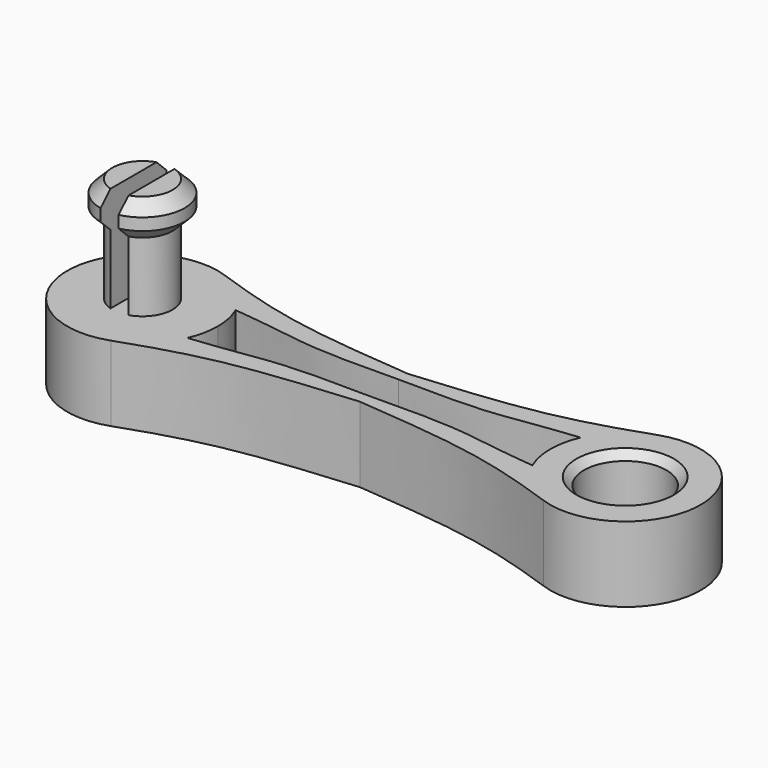
from build123d import *

# Parameters (mm, degrees)
F2_DEPTH = 6.35
F1_W     = 1.778
F1_H     = 3.048
F1_H_2   = 5.842
F1_W_2   = 0.762
F5_DEPTH = 12.7
F6_DEPTH = 2.54


# Not quite as in the source:
# - a pattern or mirror of a feature is missing from the dataset's text; its kind, count and spacing are read off the source's solid
# - a feature names something its author has since deleted; it is built from what else it names


with BuildPart() as f2:
    # F0 (on Top) → F2 (new body)
    with BuildSketch(Plane.XY):
        with BuildLine():
            ThreePointArc((-14.5509208863, -2.5399817128), (-14.1547428746, -1.2973564714), (-14.0208, 0))
            ThreePointArc((-14.0208, 0), (-14.1547428746, 1.2973564714), (-14.5509208863, 2.5399817128))
            ThreePointArc((-14.5509208863, 2.5399817128), (-16.0448887373, 4.6485472727), (-18.2552900028, 5.9872462328))
            ThreePointArc((-18.2552900028, 5.9872462328), (-26.7208, 0), (-18.2552900028, -5.9872462328))
            ThreePointArc((-18.2552900028, -5.9872462328), (-16.0448887373, -4.6485472727), (-14.5509208863, -2.5399817128))
        make_face()
        with BuildLine():
            ThreePointArc((-18.2552900028, 5.9872462328), (-16.0448887373, 4.6485472727), (-14.5509208863, 2.5399817128))
            add(Edge.make_bspline(
                [(0, 1.524), (-9.0764431036, 1.3546369813), (-7.8380626316, 1.8652065321), (-14.5509208863, 2.5399817128)],
                knots=[0, 0, 0, 0, 14.5863469546, 14.5863469546, 14.5863469546, 14.5863469546], degree=3))
            add(Edge.make_bspline(
                [(0, 1.524), (9.0764431036, 1.3546369813), (7.8380626316, 1.8652065321), (14.5509208863, 2.5399817128)],
                knots=[0, 0, 0, 0, 14.5863469546, 14.5863469546, 14.5863469546, 14.5863469546], degree=3))
            ThreePointArc((14.5509208863, 2.5399817128), (16.0448887373, 4.6485472727), (18.2552900028, 5.9872462328))
            add(Edge.make_bspline(
                [(0, 2.54), (8.1250406802, 3.246476237), (11.4529688686, 3.5837408809), (18.2552900028, 5.9872462328)],
                knots=[0, 0, 0, 0, 18.5779202193, 18.5779202193, 18.5779202193, 18.5779202193], degree=3))
            add(Edge.make_bspline(
                [(0, 2.54), (-8.1250406802, 3.246476237), (-11.4529688686, 3.5837408809), (-18.2552900028, 5.9872462328)],
                knots=[0, 0, 0, 0, 18.5779202193, 18.5779202193, 18.5779202193, 18.5779202193], degree=3))
        make_face()
        with BuildLine():
            add(Edge.make_bspline(
                [(0, -1.524), (-9.0764431036, -1.3546369813), (-7.8380626316, -1.8652065321), (-14.5509208863, -2.5399817128)],
                knots=[0, 0, 0, 0, 14.5863469546, 14.5863469546, 14.5863469546, 14.5863469546], degree=3))
            ThreePointArc((-14.5509208863, -2.5399817128), (-16.0448887373, -4.6485472727), (-18.2552900028, -5.9872462328))
            add(Edge.make_bspline(
                [(0, -2.54), (-8.1250406802, -3.246476237), (-11.4529688686, -3.5837408809), (-18.2552900028, -5.9872462328)],
                knots=[0, 0, 0, 0, 18.5779202193, 18.5779202193, 18.5779202193, 18.5779202193], degree=3))
            add(Edge.make_bspline(
                [(0, -2.54), (8.1250406802, -3.246476237), (11.4529688686, -3.5837408809), (18.2552900028, -5.9872462328)],
                knots=[0, 0, 0, 0, 18.5779202193, 18.5779202193, 18.5779202193, 18.5779202193], degree=3))
            ThreePointArc((18.2552900028, -5.9872462328), (16.0448887373, -4.6485472727), (14.5509208863, -2.5399817128))
            add(Edge.make_bspline(
                [(0, -1.524), (9.0764431036, -1.3546369813), (7.8380626316, -1.8652065321), (14.5509208863, -2.5399817128)],
                knots=[0, 0, 0, 0, 14.5863469546, 14.5863469546, 14.5863469546, 14.5863469546], degree=3))
        make_face()
    extrude(amount=F2_DEPTH)

    # F2_copies: F2 across plane


with BuildPart() as f2_1:
    add(f2.part)
    add(f2.part.mirror(Plane(origin=(0, 0, 0), x_dir=(0, 0, 1), z_dir=(1, 0, 0))))

    # F1 (on Front) → F3 (revolve, cut)
    with BuildSketch(Plane.XZ):
        Polygon((20.344351037, 6.35), (20.344351037, 0), (24.459151037, 0), (23.824151037, 0.635), (23.824151037, 5.715), (24.459151037, 6.35), align=None)
    revolve(axis=Axis((20.344351037, 0, 3.175), (0, 0, 1)), mode=Mode.SUBTRACT)

    # F1 (on Front) → F4 (revolve)
    with BuildSketch(Plane.XZ):
        Polygon((-17.8308, 15.24), (-17.8308, 12.192), (-16.8148, 13.208), (-16.8148, 14.224), align=None)
        with Locations((-18.7198, 13.716)):
            Rectangle(F1_W, F1_H)
        with Locations((-22.0218, 13.716)):
            Rectangle(F1_W, F1_H)
        Polygon((-23.9268, 13.208), (-22.9108, 12.192), (-22.9108, 15.24), (-23.9268, 14.224), align=None)
        with Locations((-22.0218, 9.271)):
            Rectangle(F1_W, F1_H_2)
        with Locations((-18.7198, 9.271)):
            Rectangle(F1_W, F1_H_2)
    revolve(axis=Axis((-20.3708, 0, 10.795), (0, 0, 1)))

    # F1 (on Front) → F5 (cut, symmetric)
    with BuildSketch(Plane.XZ):
        with Locations((-19.9898, 13.716)):
            Rectangle(F1_W_2, F1_H)
        with Locations((-20.7518, 13.716)):
            Rectangle(F1_W_2, F1_H)
        with Locations((-19.9898, 9.271)):
            Rectangle(F1_W_2, F1_H_2)
        with Locations((-20.7518, 9.271)):
            Rectangle(F1_W_2, F1_H_2)
    extrude(amount=F5_DEPTH, both=True, mode=Mode.SUBTRACT)

    # F0 (on Top) → F6 (join)
    with BuildSketch(Plane.XY):
        with BuildLine():
            ThreePointArc((-14.5509208863, 2.5399817128), (-14.1547428746, 1.2973564714), (-14.0208, 0))
            ThreePointArc((-14.0208, 0), (-14.1547428746, -1.2973564714), (-14.5509208863, -2.5399817128))
            add(Edge.make_bspline(
                [(0, -1.524), (-9.0764431036, -1.3546369813), (-7.8380626316, -1.8652065321), (-14.5509208863, -2.5399817128)],
                knots=[0, 0, 0, 0, 14.5863469546, 14.5863469546, 14.5863469546, 14.5863469546], degree=3))
            add(Edge.make_bspline(
                [(0, -1.524), (9.0764431036, -1.3546369813), (7.8380626316, -1.8652065321), (14.5509208863, -2.5399817128)],
                knots=[0, 0, 0, 0, 14.5863469546, 14.5863469546, 14.5863469546, 14.5863469546], degree=3))
            ThreePointArc((14.5509208863, -2.5399817128), (14.0208, 0), (14.5509208863, 2.5399817128))
            add(Edge.make_bspline(
                [(0, 1.524), (9.0764431036, 1.3546369813), (7.8380626316, 1.8652065321), (14.5509208863, 2.5399817128)],
                knots=[0, 0, 0, 0, 14.5863469546, 14.5863469546, 14.5863469546, 14.5863469546], degree=3))
            add(Edge.make_bspline(
                [(0, 1.524), (-9.0764431036, 1.3546369813), (-7.8380626316, 1.8652065321), (-14.5509208863, 2.5399817128)],
                knots=[0, 0, 0, 0, 14.5863469546, 14.5863469546, 14.5863469546, 14.5863469546], degree=3))
        make_face()
    extrude(amount=F6_DEPTH)


solid = f2_1.part
